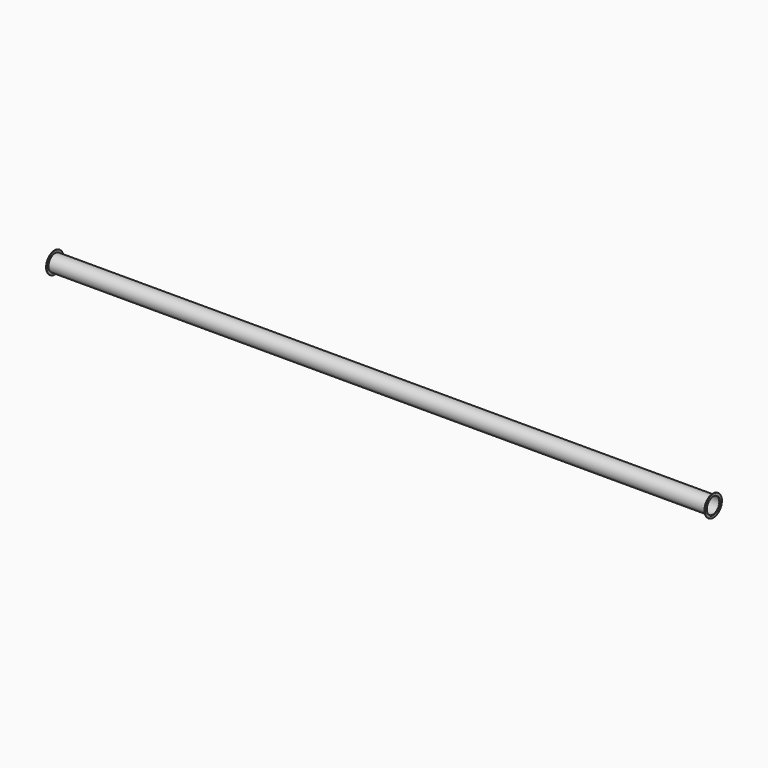
from build123d import *

# Parameters (mm, degrees)
F0_W     = 6192
F0_H     = 3
F2_R     = 100
F2_R_2   = 78
F2_R_3   = 75
F3_DEPTH = 5
F4_R     = 100
F4_R_2   = 78
F5_DEPTH = 5


with BuildPart() as f1:
    # F0 (on Front) → F1 (revolve)
    with BuildSketch(Plane.XZ):
        with Locations((-3096, 76.5)):
            Rectangle(F0_W, F0_H)
    revolve(axis=Axis((-3096, 0, 0), (-1, 0, 0)))


with BuildPart() as f3:
    # F2 (on face) → F3 (new body)
    with BuildSketch(Plane(origin=(-6192, 0, 0), x_dir=(0, -1, 0), z_dir=(-1, 0, 0))):
        Circle(F2_R)
        Circle(F2_R_2, mode=Mode.SUBTRACT)
        Circle(F2_R_2)
        Circle(F2_R_3, mode=Mode.SUBTRACT)
    extrude(amount=F3_DEPTH)


with BuildPart() as f5:
    # F4 (on face) → F5 (new body)
    with BuildSketch(Plane.YZ):
        Circle(F4_R)
        Circle(F4_R_2, mode=Mode.SUBTRACT)
    extrude(amount=F5_DEPTH)


solid = Compound([f1.part, f3.part, f5.part])
